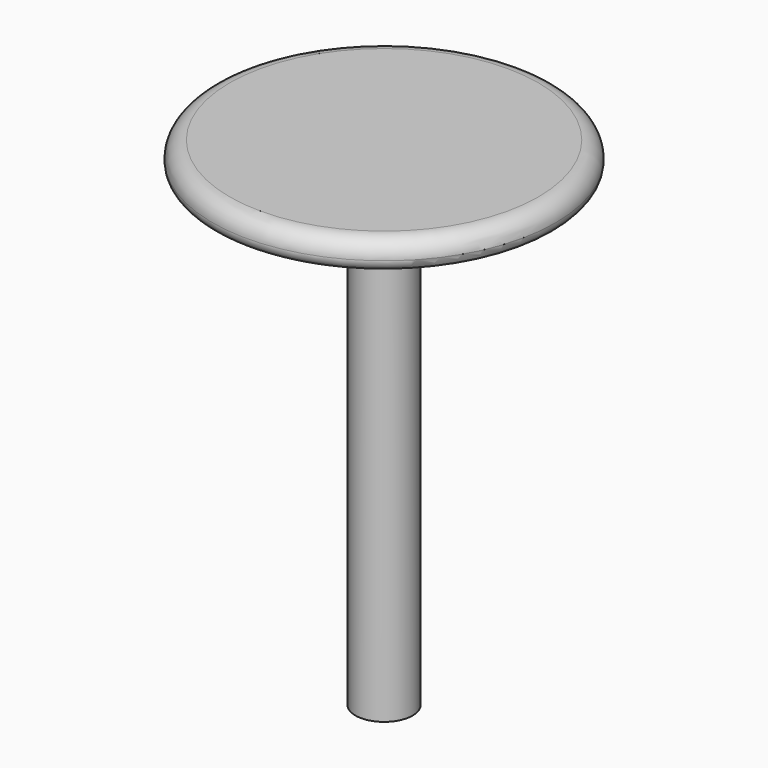
from build123d import *

# Parameters (mm, degrees)
F0_R     = 30
F1_DEPTH = 5
F2_R     = 3
F3_R     = 1.99999
F4_R     = 5
F5_DEPTH = 82


# Not quite as in the source:
# - a fillet or chamfer is up to 0.001 mm smaller than in the source, because OpenCascade refuses the exact size


with BuildPart() as f1:
    # F0 (on Top) → F1 (new body)
    with BuildSketch(Plane.XY):
        Circle(F0_R)
    extrude(amount=F1_DEPTH)

    # F2
    f2_edges = [f1.edges().sort_by_distance(p)[0] for p in [
        (-30, 0, 5),
    ]]
    fillet(f2_edges, radius=F2_R)

    # F3 (radius 2 in the source; OpenCascade refuses exactly that, so slightly less here)
    f3_edges = [f1.edges().sort_by_distance(p)[0] for p in [
        (-30, 0, 0),
    ]]
    fillet(f3_edges, radius=F3_R)

    # F4 (on face) → F5 (join)
    with BuildSketch(Plane(origin=(0, 0, 0), x_dir=(1, 0, 0), z_dir=(0, 0, -1))):
        Circle(F4_R)
    extrude(amount=F5_DEPTH)


solid = f1.part
